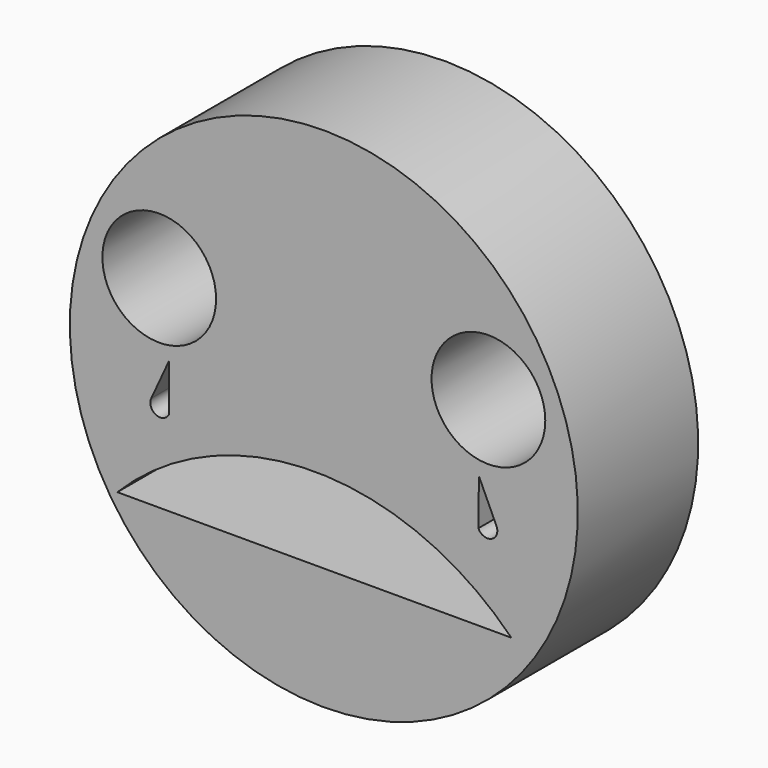
from build123d import *

# Parameters (mm, degrees)
F0_R     = 4.3187243864
F1_DEPTH = 11.43
F4_DEPTH = 25.4
F6_DEPTH = 25.4


# Not quite as in the source:
# - a pattern or mirror of a feature is missing from the dataset's text; its kind, count and spacing are read off the source's solid
# - the program builds the solid bodies; features that only make, move or delete a surface that nothing else refers to are left out


with BuildPart() as f1:
    # F0 (on Front) → F1 (new body)
    with BuildSketch(Plane.XZ):
        with BuildLine():
            ThreePointArc((-16.2297749531, -10.4286198462), (-16.1842309709, -10.4991606713), (-16.1383803934, -10.5695025995))
            ThreePointArc((-16.1383803934, -10.5695025995), (5.5149003864, -18.4864161116), (19.2914931232, 0))
            ThreePointArc((19.2914931232, 0), (-5.4343865811, 18.5102444449), (-16.2297749531, -10.4286198462))
        make_face()
        with Locations((-12.5015638769, 5.341576878)):
            Circle(F0_R, mode=Mode.SUBTRACT)
        with Locations((12.5015638769, 5.341576878)):
            Circle(F0_R, mode=Mode.SUBTRACT)
    extrude(amount=F1_DEPTH)

    # F2 (on Front) → F4 (cut)
    with BuildSketch(Plane.XZ):
        with BuildLine():
            Line((-15.6837776303, -10.0077530369), (14.2410276458, -10.0077530369))
            ThreePointArc((14.2410276458, -10.0077530369), (-0.7213749923, -3.7564431571), (-15.6837776303, -10.0077530369))
        make_face()
    extrude(amount=F4_DEPTH, mode=Mode.SUBTRACT)

    # F5 (on face) → F6 (cut)
    with BuildSketch(Plane.XZ.offset(11.43)):
        with BuildLine():
            Line((-11.7404377088, -3.5014220048), (-11.7787355557, 0))
            Line((-11.7787355557, 0), (-13.1083335727, -2.8944755904))
            ThreePointArc((-13.1083335727, -2.8944755904), (-12.7318294924, -3.8908455066), (-11.7404377088, -3.5014220048))
        make_face()
    f6 = extrude(amount=-F6_DEPTH, mode=Mode.SUBTRACT)

    # F6_copies: F6 across plane
    add(f6.mirror(Plane(origin=(0, 0, 0), x_dir=(0, 0, 1), z_dir=(1, 0, 0))), mode=Mode.SUBTRACT)


solid = f1.part
